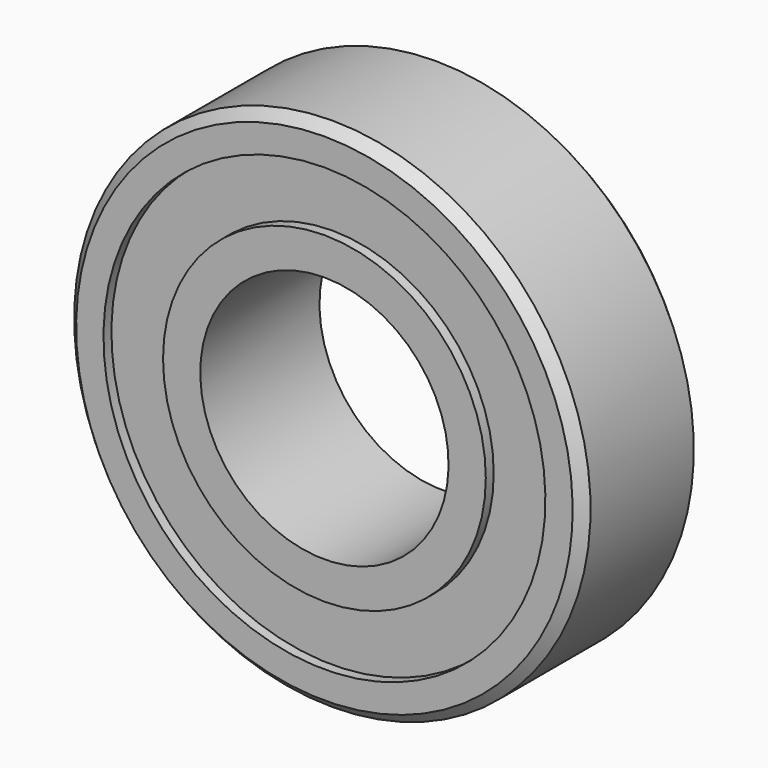
from build123d import *

# Parameters (mm, degrees)
F3_SIZE         = 1
F4_COPIES_COUNT = 12
F1_W            = 1
F1_H            = 1
F1_H_2          = 6


# Not quite as in the source:
# - a pattern or mirror of a feature is missing from the dataset's text; its kind, count and spacing are read off the source's solid
# - a feature names something its author has since deleted; it is built from what else it names


with BuildPart() as f2:
    # F1 (on Right) → F2 (revolve)
    with BuildSketch(Plane.YZ):
        with BuildLine():
            Line((7.5, 26), (-7.5, 26))
            Line((-7.5, 26), (-7.5, 22.25))
            Line((-7.5, 22.25), (-6.5, 22.25))
            Line((-6.5, 22.25), (-6.5, 23.25))
            Line((-6.5, 23.25), (-5.5, 23.25))
            Line((-5.5, 23.25), (-5.5, 22.25))
            Line((-5.5, 22.25), (-2.6457513111, 22.25))
            ThreePointArc((-2.6457513111, 22.25), (0, 23.25), (2.6457513111, 22.25))
            Line((2.6457513111, 22.25), (7.5, 22.25))
            Line((7.5, 22.25), (7.5, 26))
        make_face()
    revolve(axis=Axis((0, 0, 0), (0, 1, 0)))

    # F3
    f3_edges = [f2.edges().sort_by_distance(p)[0] for p in [
        (0, 7.5, -26),
        (0, -7.5, -26),
    ]]
    chamfer(f3_edges, length=F3_SIZE)



with BuildPart() as f2b:
    # F1 (on Right) → F2, piece 2 (revolve)
    with BuildSketch(Plane.YZ):
        with BuildLine():
            Line((-6.5, 16.25), (-7.5, 16.25))
            Line((-7.5, 16.25), (-7.5, 12.5))
            Line((-7.5, 12.5), (7.5, 12.5))
            Line((7.5, 12.5), (7.5, 16.25))
            Line((7.5, 16.25), (2.6457513111, 16.25))
            ThreePointArc((2.6457513111, 16.25), (0, 15.25), (-2.6457513111, 16.25))
            Line((-2.6457513111, 16.25), (-5.5, 16.25))
            Line((-5.5, 16.25), (-5.5, 15.25))
            Line((-5.5, 15.25), (-6.5, 15.25))
            Line((-6.5, 15.25), (-6.5, 16.25))
        make_face()
    revolve(axis=Axis((0, 0, 0), (0, 1, 0)))


with BuildPart() as f4:
    # F1 (on Right) → F4 (revolve)
    with BuildSketch(Plane.YZ):
        with BuildLine():
            ThreePointArc((4, 19.25), (3.6457513111, 20.8957513111), (2.6457513111, 22.25))
            Line((2.6457513111, 22.25), (-2.6457513111, 22.25))
            ThreePointArc((-2.6457513111, 22.25), (-3.6457513111, 20.8957513111), (-4, 19.25))
            Line((-4, 19.25), (4, 19.25))
        make_face()
        with BuildLine():
            Line((-2.6457513111, 22.25), (2.6457513111, 22.25))
            ThreePointArc((2.6457513111, 22.25), (0, 23.25), (-2.6457513111, 22.25))
        make_face()
    revolve(axis=Axis((0, 0.4880432971, 19.25), (0, 1, 0)))


with BuildPart() as f4_copies_1:
    # F4_copies: instance of F4
    add(f4.part.rotate(Axis((0, 0, 0), (0, 1, 0)), 1 * 360 / F4_COPIES_COUNT))


with BuildPart() as f4_copies_2:
    # F4_copies: instance of F4
    add(f4.part.rotate(Axis((0, 0, 0), (0, 1, 0)), 2 * 360 / F4_COPIES_COUNT))


with BuildPart() as f4_copies_3:
    # F4_copies: instance of F4
    add(f4.part.rotate(Axis((0, 0, 0), (0, 1, 0)), 3 * 360 / F4_COPIES_COUNT))


with BuildPart() as f4_copies_4:
    # F4_copies: instance of F4
    add(f4.part.rotate(Axis((0, 0, 0), (0, 1, 0)), 4 * 360 / F4_COPIES_COUNT))


with BuildPart() as f4_copies_5:
    # F4_copies: instance of F4
    add(f4.part.rotate(Axis((0, 0, 0), (0, 1, 0)), 5 * 360 / F4_COPIES_COUNT))


with BuildPart() as f4_copies_6:
    # F4_copies: instance of F4
    add(f4.part.rotate(Axis((0, 0, 0), (0, 1, 0)), 6 * 360 / F4_COPIES_COUNT))


with BuildPart() as f4_copies_7:
    # F4_copies: instance of F4
    add(f4.part.rotate(Axis((0, 0, 0), (0, 1, 0)), 7 * 360 / F4_COPIES_COUNT))


with BuildPart() as f4_copies_8:
    # F4_copies: instance of F4
    add(f4.part.rotate(Axis((0, 0, 0), (0, 1, 0)), 8 * 360 / F4_COPIES_COUNT))


with BuildPart() as f4_copies_9:
    # F4_copies: instance of F4
    add(f4.part.rotate(Axis((0, 0, 0), (0, 1, 0)), 9 * 360 / F4_COPIES_COUNT))


with BuildPart() as f4_copies_10:
    # F4_copies: instance of F4
    add(f4.part.rotate(Axis((0, 0, 0), (0, 1, 0)), 10 * 360 / F4_COPIES_COUNT))


with BuildPart() as f4_copies_11:
    # F4_copies: instance of F4
    add(f4.part.rotate(Axis((0, 0, 0), (0, 1, 0)), 11 * 360 / F4_COPIES_COUNT))


with BuildPart() as f2_1:
    add(f2.part)

    add(f2b.part)  # F5 merges F2b
    # F1 (on Right) → F5 (revolve)
    with BuildSketch(Plane.YZ):
        with Locations((-6, 22.75)):
            Rectangle(F1_W, F1_H)
        with Locations((-6, 19.25)):
            Rectangle(F1_W, F1_H_2)
        with Locations((-6, 15.75)):
            Rectangle(F1_W, F1_H)
    revolve(axis=Axis((0, 0, 0), (0, 1, 0)))

    # F6: union F4
    add(f4.part)


solid = Compound([f4_copies_1.part, f4_copies_2.part, f4_copies_3.part, f4_copies_4.part, f4_copies_5.part, f4_copies_6.part, f4_copies_7.part, f4_copies_8.part, f4_copies_9.part, f4_copies_10.part, f4_copies_11.part, f2_1.part])
